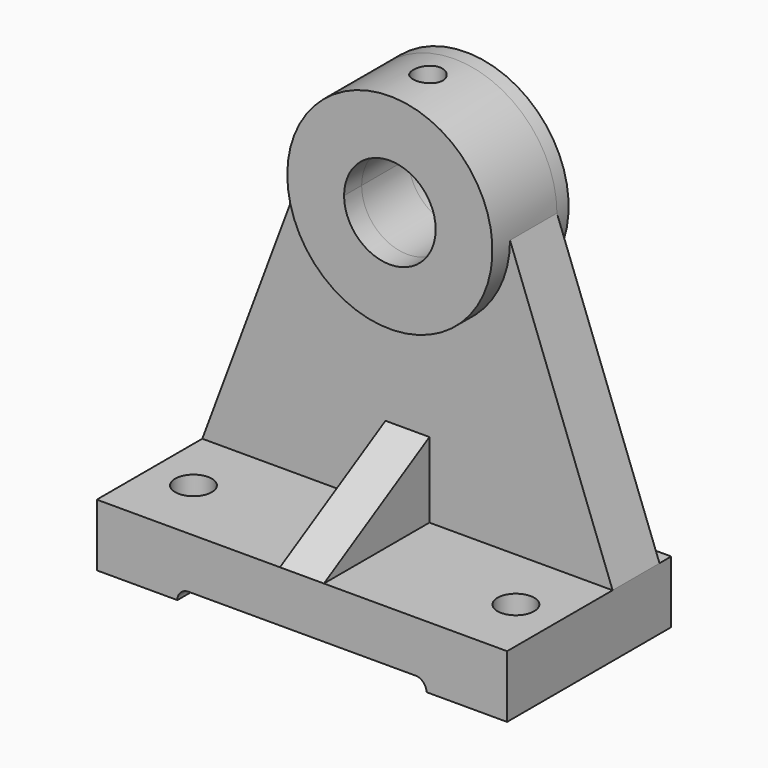
from build123d import *

# Parameters (mm, degrees)
F1_DEPTH       = 112
F2_W           = 4
F2_H           = 75
F3_DEPTH       = 112.001
F5_DEPTH       = 50
F7_DEPTH       = 50
F9_DEPTH       = 25
F8_R           = 12.5
F10_DEPTH      = 4
F10_DEPTH_BACK = 22
F12_W          = 68
F12_H          = 3
F13_DEPTH      = 56.001
F14_R          = 5
F15_DEPTH      = 25
F16_R          = 4
F17_DEPTH      = 117.001
F18_R          = 4
F19_DEPTH      = 80
F11_R          = 12.5
F20_DEPTH      = 25
F20_DEPTH_BACK = 25
F21_R          = 2.99999


# Not quite as in the source:
# - a fillet or chamfer is up to 0.001 mm smaller than in the source, because OpenCascade refuses the exact size
# - a feature names something its author has since deleted; it is built from what else it names


with BuildPart() as f1:
    # F0 (on Right) → F1 (new body)
    with BuildSketch(Plane.YZ):
        Polygon((-56, 0), (0, 0), (0, 49), (0, 92), (-20, 92), (-20, 37.5714285714), (-56, 17), align=None)
    extrude(amount=F1_DEPTH)

    # F2 (on face) → F3 (cut, through all)
    with BuildSketch(Plane.YZ.offset(112)):
        with Locations((-2, 54.5)):
            Rectangle(F2_W, F2_H)
    extrude(amount=-F3_DEPTH, mode=Mode.SUBTRACT)

    # F4 (on face) → F5 (cut)
    with BuildSketch(Plane.YZ.offset(112)):
        Polygon((-20, 37.5714285714), (-56, 17), (-20, 17), align=None)
    extrude(amount=-F5_DEPTH, mode=Mode.SUBTRACT)

    # F6 (on face) → F7 (cut)
    with BuildSketch(Plane(origin=(0, 0, 0), x_dir=(0, -1, 0), z_dir=(-1, 0, 0))):
        Polygon((20, 17), (56, 17), (20, 37.5714285714), align=None)
    extrude(amount=-F7_DEPTH, mode=Mode.SUBTRACT)

    # F8 (on face) → F9 (cut)
    with BuildSketch(Plane(origin=(0, -4, 0), x_dir=(-1, 0, 0), z_dir=(0, 1, 0))):
        Polygon((-112, 17), (-84, 92), (-112, 92), align=None)
        Polygon((0, 92), (-28, 92), (0, 17), align=None)
    extrude(amount=-F9_DEPTH, mode=Mode.SUBTRACT)

    # F8 (on face) → F10 (join, two sides)
    with BuildSketch(Plane(origin=(0, -4, 0), x_dir=(-1, 0, 0), z_dir=(0, 1, 0))) as f10_sk:
        with BuildLine():
            ThreePointArc((-84, 92), (-56, 64), (-28, 92))
            ThreePointArc((-28, 92), (-56, 120), (-84, 92))
        make_face()
        with Locations((-56, 92)):
            Circle(F8_R, mode=Mode.SUBTRACT)
    extrude(amount=F10_DEPTH)
    extrude(f10_sk.sketch, amount=-F10_DEPTH_BACK)

    # F12 (on face) → F13 (cut, through all)
    with BuildSketch(Plane.XZ.offset(56)):
        with Locations((56, 1.5)):
            Rectangle(F12_W, F12_H)
    extrude(amount=-F13_DEPTH, mode=Mode.SUBTRACT)

    # F14 (on face) → F15 (cut)
    with BuildSketch(Plane.XY.offset(17)):
        with Locations((12, -38)):
            Circle(F14_R)
        with Locations((100, -38)):
            Circle(F14_R)
    extrude(amount=-F15_DEPTH, mode=Mode.SUBTRACT)

    # F16 (on face) → F17 (cut, through all)
    with BuildSketch(Plane(origin=(0, 0, 3), x_dir=(1, 0, 0), z_dir=(0, 0, -1))):
        with Locations((56, 13)):
            Circle(F16_R)
    extrude(amount=-F17_DEPTH, mode=Mode.SUBTRACT)

    # F18 (on face) → F19 (join)
    with BuildSketch(Plane(origin=(0, 0, 3), x_dir=(1, 0, 0), z_dir=(0, 0, -1))):
        with Locations((56, 13)):
            Circle(F18_R)
    extrude(amount=-F19_DEPTH)

    # F11 (on face) → F20 (cut, two sides)
    with BuildSketch(Plane.XZ.offset(20)) as f20_sk:
        with Locations((56, 92)):
            Circle(F11_R)
    extrude(amount=-F20_DEPTH, mode=Mode.SUBTRACT)
    extrude(f20_sk.sketch, amount=F20_DEPTH_BACK, mode=Mode.SUBTRACT)

    # F21 (radius 3 in the source; OpenCascade refuses exactly that, so slightly less here)
    f21_edges = [f1.edges().sort_by_distance(p)[0] for p in [
        (22, -28, 3),
        (90, -28, 3),
    ]]
    fillet(f21_edges, radius=F21_R)


solid = f1.part
